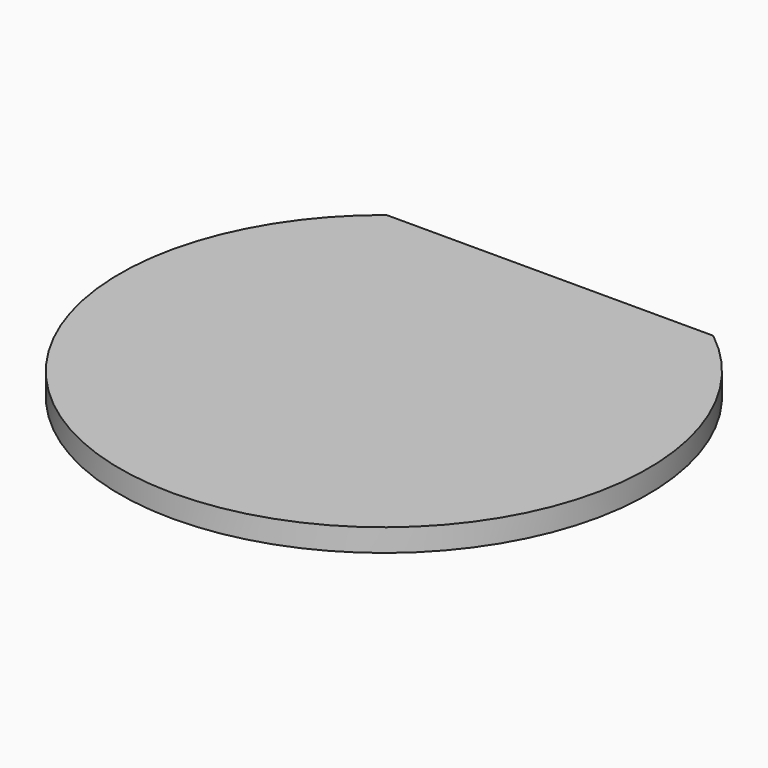
from build123d import *

# Parameters (mm, degrees)
F0_R     = 70
F1_DEPTH = 6
F4_DEPTH = 6


with BuildPart() as f1:
    # F0 (on Top) → F1 (new body)
    with BuildSketch(Plane.XY):
        Circle(F0_R)
    extrude(amount=-F1_DEPTH)

    # F3 (on face) → F4 (cut)
    with BuildSketch(Plane(origin=(0, 0, -6), x_dir=(1, 0, 0), z_dir=(0, 0, -1))):
        with BuildLine():
            Line((43.3012701892, -55), (0, -55))
            Line((0, -55), (-43.3012701892, -55))
            ThreePointArc((-43.3012701892, -55), (0, -70), (43.3012701892, -55))
        make_face()
    extrude(amount=-F4_DEPTH, mode=Mode.SUBTRACT)


solid = f1.part
